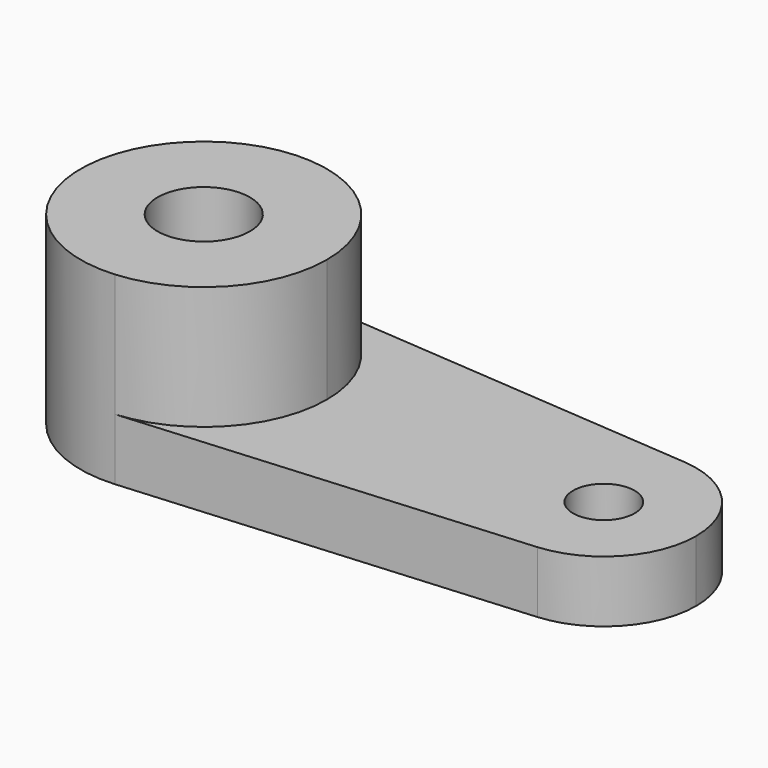
from build123d import *

# Parameters (mm, degrees)
F0_R     = 9.525
F1_DEPTH = 38.1
F0_R_2   = 6.35
F2_DEPTH = 12.7


# Not quite as in the source:
# - a feature of the source that left no trace in its solid (it failed there, or was rolled back) is left out


with BuildPart() as f1:
    # F0 (on Top) → F1 (new body)
    with BuildSketch(Plane.XY):
        with BuildLine():
            ThreePointArc((1.9538461538, -25.3247405753), (18.6385043969, -17.2559020004), (25.4, 0))
            ThreePointArc((25.4, 0), (18.6385043969, 17.2559020004), (1.9538461538, 25.3247405753))
            ThreePointArc((1.9538461538, 25.3247405753), (-25.4, 0), (1.9538461538, -25.3247405753))
        make_face()
        Circle(F0_R, mode=Mode.SUBTRACT)
    extrude(amount=F1_DEPTH)

    # F0 (on Top) → F2 (join)
    with BuildSketch(Plane.XY):
        with BuildLine():
            ThreePointArc((1.9538461538, -25.3247405753), (18.6385043969, -17.2559020004), (25.4, 0))
            ThreePointArc((25.4, 0), (18.6385043969, 17.2559020004), (1.9538461538, 25.3247405753))
            ThreePointArc((1.9538461538, 25.3247405753), (-25.4, 0), (1.9538461538, -25.3247405753))
        make_face()
        Circle(F0_R, mode=Mode.SUBTRACT)
        with BuildLine():
            ThreePointArc((1.9538461538, 25.3247405753), (18.6385043969, 17.2559020004), (25.4, 0))
            ThreePointArc((25.4, 0), (18.6385043969, -17.2559020004), (1.9538461538, -25.3247405753))
            Line((1.9538461538, -25.3247405753), (84.0153846154, -18.9935554315))
            ThreePointArc((84.0153846154, -18.9935554315), (63.5, 0), (84.0153846154, 18.9935554315))
            Line((84.0153846154, 18.9935554315), (1.9538461538, 25.3247405753))
        make_face()
        with BuildLine():
            ThreePointArc((101.6, 0), (96.5288782977, 12.9419265003), (84.0153846154, 18.9935554315))
            ThreePointArc((84.0153846154, 18.9935554315), (63.5, 0), (84.0153846154, -18.9935554315))
            ThreePointArc((84.0153846154, -18.9935554315), (96.5288782977, -12.9419265003), (101.6, 0))
        make_face()
        with Locations((82.55, 0)):
            Circle(F0_R_2, mode=Mode.SUBTRACT)
    extrude(amount=F2_DEPTH)


solid = f1.part
